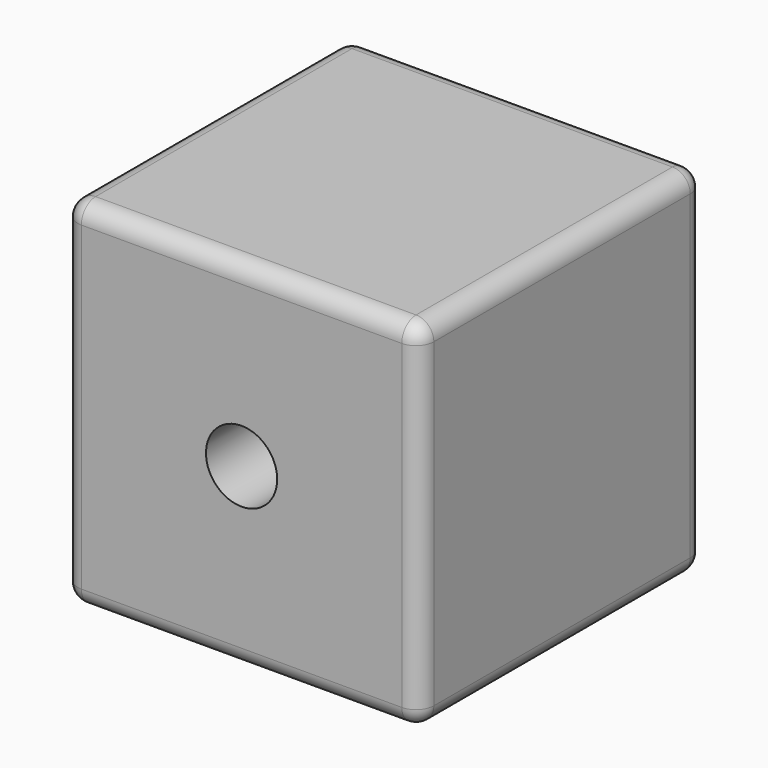
from build123d import *

# Parameters (mm, degrees)
F0_W     = 100
F0_H     = 100
F1_DEPTH = 100
F2_R     = 5
F3_DEPTH = 100
F5_R     = 10
F6_DEPTH = 25
F7_R     = 5


# Not quite as in the source:
# - a pattern or mirror of a feature is missing from the dataset's text; its kind, count and spacing are read off the source's solid


with BuildPart() as f1:
    # F0 (on Front) → F1 (new body)
    with BuildSketch(Plane.XZ):
        with Locations((50, 50)):
            Rectangle(F0_W, F0_H)
    extrude(amount=F1_DEPTH)

    # F2 (on face) → F3 (cut)
    with BuildSketch(Plane.XZ.offset(100)):
        with Locations((50, 50)):
            Circle(F2_R)
    extrude(amount=-F3_DEPTH, mode=Mode.SUBTRACT)

    # F5 (on face) → F6 (cut)
    with BuildSketch(Plane.XZ.offset(100)):
        with Locations((50, 50)):
            Circle(F5_R)
    f6 = extrude(amount=-F6_DEPTH, mode=Mode.SUBTRACT)

    # F6_copies: F6 across plane
    add(f6.mirror(Plane.ZX.offset(-50)), mode=Mode.SUBTRACT)

    # F7
    f7_edges = [f1.edges().sort_by_distance(p)[0] for p in [
        (0, -50, 100),
        (50, -100, 100),
        (100, -50, 100),
        (50, 0, 100),
        (0, -100, 50),
        (50, -100, 0),
        (100, -100, 50),
        (100, -50, 0),
        (100, 0, 50),
        (50, 0, 0),
        (0, 0, 50),
        (0, -50, 0),
    ]]
    fillet(f7_edges, radius=F7_R)


solid = f1.part
